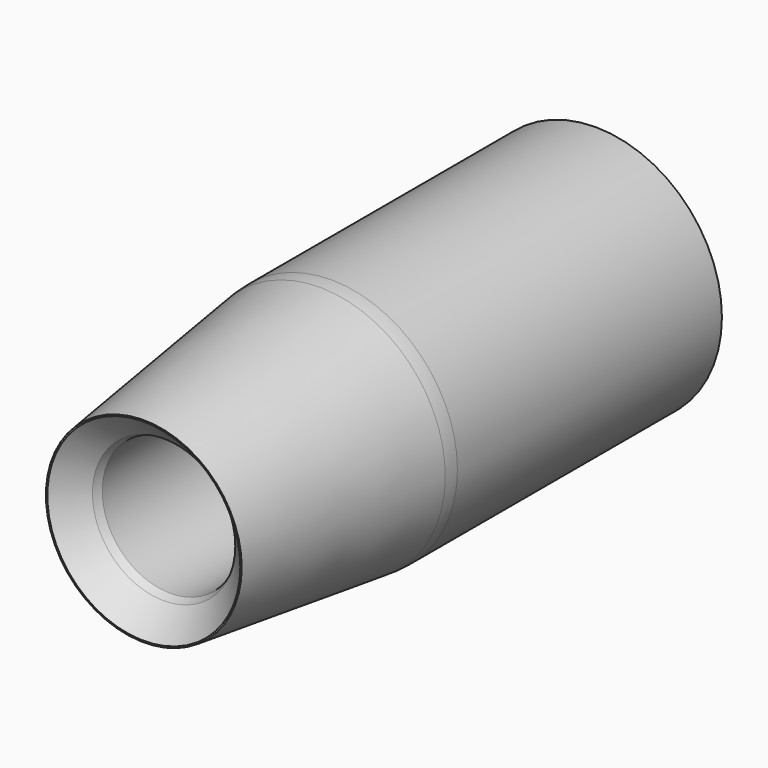
from build123d import *

# Parameters (mm, degrees)
F0_R     = 22.25
F1_DEPTH = 100
F2_R     = 20.75
F3_DEPTH = 60
F4_R     = 12
F5_DEPTH = 191.6
F6_SIZE2 = 40
F6_SIZE  = 5
F7_SIZE  = 5
F8_R     = 20


# Not quite as in the source:
# - a fillet or chamfer that OpenCascade refuses, or shapes differently, is made with other operations: its cross-section is extruded or revolved along the edge and cut away or added


with BuildPart() as f1:
    # F0 (on Front) → F1 (new body)
    with BuildSketch(Plane.XZ):
        Circle(F0_R)
    extrude(amount=F1_DEPTH)

    # F2 (on Front) → F3 (cut)
    with BuildSketch(Plane.XZ):
        Circle(F2_R)
    extrude(amount=F3_DEPTH, mode=Mode.SUBTRACT)

    # F4 (on Front) → F5 (cut)
    with BuildSketch(Plane.XZ):
        Circle(F4_R)
    extrude(amount=F5_DEPTH, mode=Mode.SUBTRACT)

    # F6
    f6_edges = [f1.edges().sort_by_distance(p)[0] for p in [
        (-22.25, -100, 0),
    ]]
    f6_side = f1.faces().sort_by_distance((-21.620675, -100, 0))[0]
    chamfer(f6_edges, length=F6_SIZE, length2=F6_SIZE2, reference=f6_side)

    # F7
    f7_edges = [f1.edges().sort_by_distance(p)[0] for p in [
        (-20.75, -60, 0),
        (-12, -100, 0),
    ]]
    chamfer(f7_edges, length=F7_SIZE)

    # F8
    f8_edges = [f1.edges().sort_by_distance(p)[0] for p in [
        (-22.25, -60, 0),
    ]]
    fillet(f8_edges, radius=F8_R)

    # F9: chamfer of 2 on 2 edges, made by hand

    # F9_s1 → F9_t2 (revolve, cut)
    with BuildSketch(Plane.XY):
        with BuildLine():
            Line((22.8065685425, 0.0565685425), (20.6934314575, -2.0565685425))
            Line((20.6934314575, -2.0565685425), (20.6534314575, -2.0565685425))
            ThreePointArc((20.6534314575, -2.0565685425), (20.71, -1.0282842712), (20.71, 0))
            Line((20.71, 0), (20.75, 0.04))
            ThreePointArc((20.75, 0.04), (21.7782842712, 0.04), (22.8065685425, 0.0965685425))
            Line((22.8065685425, 0.0965685425), (22.8065685425, 0.0565685425))
        make_face()
    revolve(axis=Axis((0, 0, 0), (0, -1, 0)), mode=Mode.SUBTRACT)

    # F9_s3 → F9_t4 (revolve, cut)
    with BuildSketch(Plane.XY):
        with BuildLine():
            Line((12.6164011122, -95.6596968002), (11.9693853254, -94.0976625127))
            Line((11.9693853254, -94.0976625127), (11.9293853254, -94.0976625127))
            ThreePointArc((11.9293853254, -94.0976625127), (11.96, -94.5488312563), (11.96, -95))
            Line((11.96, -95), (11.9717157288, -95.0282842712))
            ThreePointArc((11.9717157288, -95.0282842712), (12.2907402069, -95.3473087494), (12.588116841, -95.6879810715))
            Line((12.588116841, -95.6879810715), (12.6164011122, -95.6596968002))
        make_face()
    revolve(axis=Axis((0, -95, 0), (0, 1, 0)), mode=Mode.SUBTRACT)


solid = f1.part
